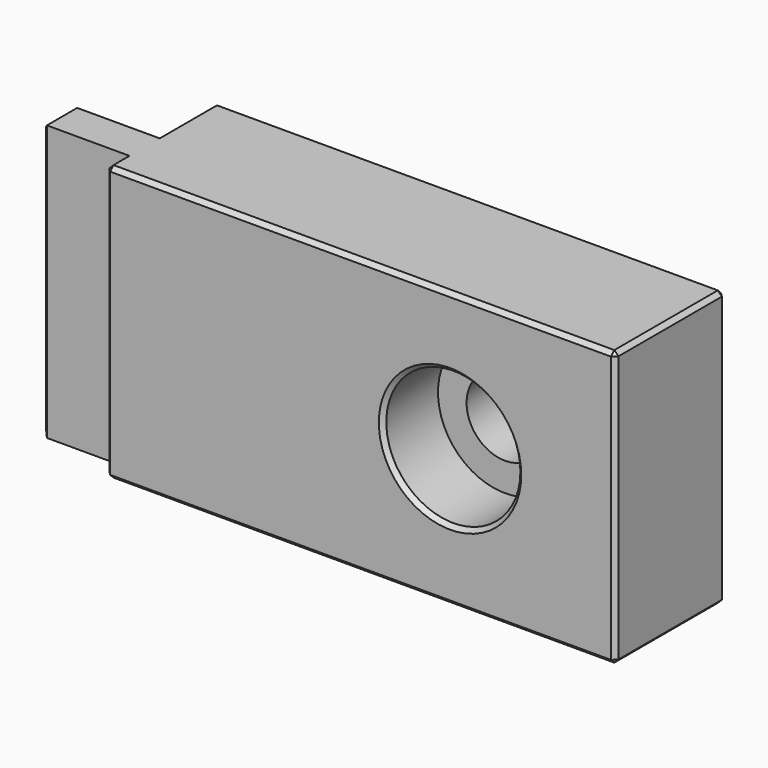
from build123d import *

# Parameters (mm, degrees)
F0_W           = 37
F0_H           = 20
F1_DEPTH       = 10
F2_D           = 5.6
F2_CBORE_D     = 9.75
F2_CBORE_DEPTH = 5
F3_W           = 2.75
F3_H           = 20
F4_DEPTH       = 6
F5_SIZE        = 0.3


with BuildPart() as f1:
    # F0 (on Front) → F1 (new body)
    with BuildSketch(Plane.XZ):
        Rectangle(F0_W, F0_H)
    extrude(amount=-F1_DEPTH)

    # F2 (through all)
    with Locations(Plane.XZ):
        with Locations((6.5, 0)):
            CounterBoreHole(F2_D / 2, F2_CBORE_D / 2, F2_CBORE_DEPTH)

    # F3 (on face) → F4 (join)
    with BuildSketch(Plane(origin=(-18.5, 0, 0), x_dir=(0, -1, 0), z_dir=(-1, 0, 0))):
        with Locations((-3.125, 0)):
            Rectangle(F3_W, F3_H)
    extrude(amount=F4_DEPTH)

    # F5
    f5_edges = [f1.edges().sort_by_distance(p)[0] for p in [
        (0, 0, 10),
        (-18.5, 0, 0),
        (0, 0, -10),
        (18.5, 0, 0),
        (18.5, 5, -10),
        (18.5, 5, 10),
        (-18.5, 0.875, -10),
        (-18.5, 7.25, -10),
        (-24.5, 3.125, -10),
        (-24.5, 3.125, 10),
        (-18.5, 0.875, 10),
        (-18.5, 7.25, 10),
        (-24.5, 1.75, 0),
        (-24.5, 4.5, 0),
        (-18.5, 10, 0),
        (0, 10, 10),
        (0, 10, -10),
        (18.5, 10, 0),
        (1.625, 0, 0),
    ]]
    chamfer(f5_edges, length=F5_SIZE)


solid = f1.part
